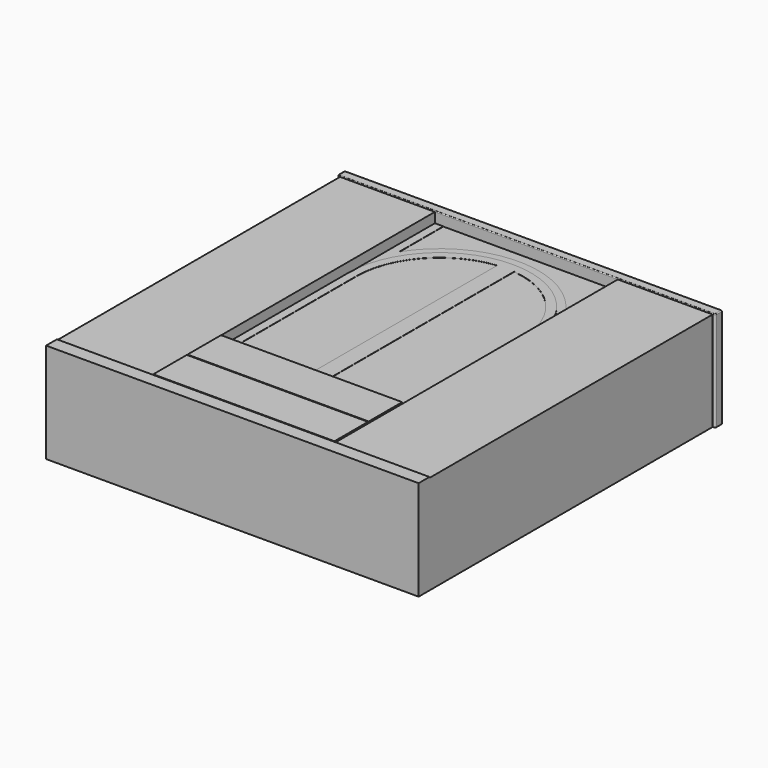
from build123d import *

# Parameters (mm, degrees)
F0_W     = 1070
F0_H     = 247.5
F0_W_2   = 440
F0_H_2   = 876.6265964508
F1_DEPTH = 590
F2_R     = 10
F3_DEPTH = 65
F4_DEPTH = 64
F5_DEPTH = 62
F6_DEPTH = 63
F7_DEPTH = 5
F8_R     = 4.99999
F9_DEPTH = 18


# Not quite as in the source:
# - a fillet or chamfer is up to 0.001 mm smaller than in the source, because OpenCascade refuses the exact size
# - a feature of the source that left no trace in its solid (it failed there, or was rolled back) is left out


with BuildPart() as f1:
    # F0 (on Top) → F1 (new body)
    with BuildSketch(Plane.XY):
        with BuildLine():
            Line((-1640, 1530), (-1640, 1135))
            Line((-1640, 1135), (-1640, 590))
            Line((-1640, 590), (-1100, 590))
            Line((-1100, 590), (-1100, 1511.6265964508))
            Line((-1100, 1511.6265964508), (-1100, 2020))
            Line((-1100, 2020), (-1100, 2070))
            ThreePointArc((-1100, 2070), (-1481.8376618407, 1911.8376618407), (-1640, 1530))
        make_face()
        with BuildLine():
            Line((-1150, 1530), (-1150, 1511.6265964508))
            Line((-1150, 1511.6265964508), (-1150, 635))
            Line((-1150, 635), (-1590, 635))
            Line((-1590, 635), (-1590, 1511.6265964508))
            Line((-1590, 1511.6265964508), (-1590, 1530))
            ThreePointArc((-1590, 1530), (-1463.7306695895, 1858.3291031876), (-1150, 2017.4423042782))
            Line((-1150, 2017.4423042782), (-1150, 1530))
        make_face(mode=Mode.SUBTRACT)
        with BuildLine():
            Line((-560, 590), (-560, 1135))
            Line((-560, 1135), (-560, 1530))
            ThreePointArc((-560, 1530), (-644.9475295345, 1820.7357032139), (-873.0638856418, 2020))
            Line((-873.0638856418, 2020), (-1100, 2020))
            Line((-1100, 2020), (-1100, 1511.6265964508))
            Line((-1100, 1511.6265964508), (-1100, 590))
            Line((-1100, 590), (-560, 590))
        make_face()
        with BuildLine():
            Line((-1050, 635), (-1050, 1511.6265964508))
            Line((-1050, 1511.6265964508), (-1050, 1530))
            Line((-1050, 1530), (-1050, 2017.4423042782))
            ThreePointArc((-1050, 2017.4423042782), (-736.2693304105, 1858.3291031876), (-610, 1530))
            Line((-610, 1530), (-610, 1511.6265964508))
            Line((-610, 1511.6265964508), (-610, 635))
            Line((-610, 635), (-1050, 635))
        make_face(mode=Mode.SUBTRACT)
        Polygon((-560, 80), (0, 80), (0, 1135), (-560, 1135), (-560, 590), align=None)
        Polygon((-2200, 1135), (-2200, 80), (-1640, 80), (-1640, 590), (-1640, 1135), align=None)
        Polygon((-2200, 2170), (-2200, 1135), (-1640, 1135), (-1640, 1530), (-1640, 2170), align=None)
        Polygon((-560, 1135), (0, 1135), (0, 2170), (-560, 2170), (-560, 1530), align=None)
        Polygon((-1100, 80), (-560, 80), (-560, 590), (-1100, 590), (-1640, 590), (-1640, 80), align=None)
        with Locations((-1100, 208.75)):
            Rectangle(F0_W, F0_H, mode=Mode.SUBTRACT)
        with Locations((-1100, 461.25)):
            Rectangle(F0_W, F0_H, mode=Mode.SUBTRACT)
        with Locations((-830, 1073.3132982254)):
            Rectangle(F0_W_2, F0_H_2)
        with Locations((-1370, 1073.3132982254)):
            Rectangle(F0_W_2, F0_H_2)
        with Locations((-1100, 461.25)):
            Rectangle(F0_W, F0_H)
        with Locations((-1100, 208.75)):
            Rectangle(F0_W, F0_H)
        Polygon((-2200, 0), (0, 0), (0, 80), (-560, 80), (-1100, 80), (-1640, 80), (-2200, 80), align=None)
        with BuildLine():
            Line((-1590, 1511.6265964508), (-1150, 1511.6265964508))
            Line((-1150, 1511.6265964508), (-1150, 1530))
            Line((-1150, 1530), (-1150, 2017.4423042782))
            ThreePointArc((-1150, 2017.4423042782), (-1463.7306695895, 1858.3291031876), (-1590, 1530))
            Line((-1590, 1530), (-1590, 1511.6265964508))
        make_face()
        with BuildLine():
            Line((-1050, 1530), (-1050, 1511.6265964508))
            Line((-1050, 1511.6265964508), (-610, 1511.6265964508))
            Line((-610, 1511.6265964508), (-610, 1530))
            ThreePointArc((-610, 1530), (-736.2693304105, 1858.3291031876), (-1050, 2017.4423042782))
            Line((-1050, 2017.4423042782), (-1050, 1530))
        make_face()
        Polygon((-560, 2170), (0, 2170), (15, 2170), (15, 2220), (0, 2220), (-2200, 2220), (-2215, 2220), (-2215, 2170), (-2200, 2170), (-1640, 2170), (-1590, 2170), (-1100, 2170), (-610, 2170), align=None)
        with BuildLine():
            Line((-1100, 2170), (-1590, 2170))
            Line((-1590, 2170), (-1590, 1846.2193073328))
            ThreePointArc((-1590, 1846.2193073328), (-1379.000923117, 2042.1065662827), (-1100, 2113.1763458252))
            Line((-1100, 2113.1763458252), (-1100, 2170))
        make_face()
        with BuildLine():
            Line((-610, 2020), (-610, 2170))
            Line((-610, 2170), (-1100, 2170))
            Line((-1100, 2170), (-1100, 2113.1763458252))
            ThreePointArc((-1100, 2113.1763458252), (-935.1694189847, 2089.397470402), (-783.7806926672, 2020))
            Line((-783.7806926672, 2020), (-610, 2020))
        make_face()
        with BuildLine():
            Line((-1590, 2170), (-1640, 2170))
            Line((-1640, 2170), (-1640, 1530))
            ThreePointArc((-1640, 1530), (-1481.8376618407, 1911.8376618407), (-1100, 2070))
            Line((-1100, 2070), (-1100, 2113.1763458252))
            ThreePointArc((-1100, 2113.1763458252), (-1379.000923117, 2042.1065662827), (-1590, 1846.2193073328))
            Line((-1590, 1846.2193073328), (-1590, 2170))
        make_face()
        with BuildLine():
            Line((-560, 1530), (-560, 2170))
            Line((-560, 2170), (-610, 2170))
            Line((-610, 2170), (-610, 2020))
            Line((-610, 2020), (-610, 1846.2193073328))
            ThreePointArc((-610, 1846.2193073328), (-687.6320512394, 1942.3679487606), (-783.7806926672, 2020))
            Line((-783.7806926672, 2020), (-873.0638856418, 2020))
            ThreePointArc((-873.0638856418, 2020), (-644.9475295345, 1820.7357032139), (-560, 1530))
        make_face()
        with BuildLine():
            Line((-610, 1846.2193073328), (-610, 2020))
            Line((-610, 2020), (-783.7806926672, 2020))
            ThreePointArc((-783.7806926672, 2020), (-687.6320512394, 1942.3679487606), (-610, 1846.2193073328))
        make_face()
        with BuildLine():
            ThreePointArc((-1100, 2070), (-983.8104996138, 2057.3518749374), (-873.0638856418, 2020))
            Line((-873.0638856418, 2020), (-783.7806926672, 2020))
            ThreePointArc((-783.7806926672, 2020), (-935.1694189847, 2089.397470402), (-1100, 2113.1763458252))
            Line((-1100, 2113.1763458252), (-1100, 2070))
        make_face()
        with BuildLine():
            Line((-1100, 2020), (-873.0638856418, 2020))
            ThreePointArc((-873.0638856418, 2020), (-983.8104996138, 2057.3518749374), (-1100, 2070))
            Line((-1100, 2070), (-1100, 2020))
        make_face()
    extrude(amount=-F1_DEPTH)

    # F2
    f2_edges = [f1.edges().sort_by_distance(p)[0] for p in [
        (15, 2170, -295),
        (-2215, 2170, -295),
    ]]
    fillet(f2_edges, radius=F2_R)

    # F0 (on Top) → F3 (cut)
    with BuildSketch(Plane.XY):
        with BuildLine():
            Line((-1100, 2170), (-1590, 2170))
            Line((-1590, 2170), (-1590, 1846.2193073328))
            ThreePointArc((-1590, 1846.2193073328), (-1379.000923117, 2042.1065662827), (-1100, 2113.1763458252))
            Line((-1100, 2113.1763458252), (-1100, 2170))
        make_face()
        with BuildLine():
            Line((-610, 2020), (-610, 2170))
            Line((-610, 2170), (-1100, 2170))
            Line((-1100, 2170), (-1100, 2113.1763458252))
            ThreePointArc((-1100, 2113.1763458252), (-935.1694189847, 2089.397470402), (-783.7806926672, 2020))
            Line((-783.7806926672, 2020), (-610, 2020))
        make_face()
        with BuildLine():
            Line((-610, 1846.2193073328), (-610, 2020))
            Line((-610, 2020), (-783.7806926672, 2020))
            ThreePointArc((-783.7806926672, 2020), (-687.6320512394, 1942.3679487606), (-610, 1846.2193073328))
        make_face()
    extrude(amount=-F3_DEPTH, mode=Mode.SUBTRACT)

    # F0 (on Top) → F4 (cut)
    with BuildSketch(Plane.XY):
        with BuildLine():
            Line((-1590, 2170), (-1640, 2170))
            Line((-1640, 2170), (-1640, 1530))
            ThreePointArc((-1640, 1530), (-1481.8376618407, 1911.8376618407), (-1100, 2070))
            Line((-1100, 2070), (-1100, 2113.1763458252))
            ThreePointArc((-1100, 2113.1763458252), (-1379.000923117, 2042.1065662827), (-1590, 1846.2193073328))
            Line((-1590, 1846.2193073328), (-1590, 2170))
        make_face()
        with BuildLine():
            ThreePointArc((-1100, 2070), (-983.8104996138, 2057.3518749374), (-873.0638856418, 2020))
            Line((-873.0638856418, 2020), (-783.7806926672, 2020))
            ThreePointArc((-783.7806926672, 2020), (-935.1694189847, 2089.397470402), (-1100, 2113.1763458252))
            Line((-1100, 2113.1763458252), (-1100, 2070))
        make_face()
        with BuildLine():
            Line((-560, 1530), (-560, 2170))
            Line((-560, 2170), (-610, 2170))
            Line((-610, 2170), (-610, 2020))
            Line((-610, 2020), (-610, 1846.2193073328))
            ThreePointArc((-610, 1846.2193073328), (-687.6320512394, 1942.3679487606), (-783.7806926672, 2020))
            Line((-783.7806926672, 2020), (-873.0638856418, 2020))
            ThreePointArc((-873.0638856418, 2020), (-644.9475295345, 1820.7357032139), (-560, 1530))
        make_face()
    extrude(amount=-F4_DEPTH, mode=Mode.SUBTRACT)

    # F0 (on Top) → F5 (cut)
    with BuildSketch(Plane.XY):
        with BuildLine():
            Line((-1640, 1530), (-1640, 1135))
            Line((-1640, 1135), (-1640, 590))
            Line((-1640, 590), (-1100, 590))
            Line((-1100, 590), (-1100, 1511.6265964508))
            Line((-1100, 1511.6265964508), (-1100, 2020))
            Line((-1100, 2020), (-1100, 2070))
            ThreePointArc((-1100, 2070), (-1481.8376618407, 1911.8376618407), (-1640, 1530))
        make_face()
        with BuildLine():
            Line((-1150, 1530), (-1150, 1511.6265964508))
            Line((-1150, 1511.6265964508), (-1150, 635))
            Line((-1150, 635), (-1590, 635))
            Line((-1590, 635), (-1590, 1511.6265964508))
            Line((-1590, 1511.6265964508), (-1590, 1530))
            ThreePointArc((-1590, 1530), (-1463.7306695895, 1858.3291031876), (-1150, 2017.4423042782))
            Line((-1150, 2017.4423042782), (-1150, 1530))
        make_face(mode=Mode.SUBTRACT)
        with BuildLine():
            Line((-1100, 2020), (-873.0638856418, 2020))
            ThreePointArc((-873.0638856418, 2020), (-983.8104996138, 2057.3518749374), (-1100, 2070))
            Line((-1100, 2070), (-1100, 2020))
        make_face()
        with BuildLine():
            Line((-560, 590), (-560, 1135))
            Line((-560, 1135), (-560, 1530))
            ThreePointArc((-560, 1530), (-644.9475295345, 1820.7357032139), (-873.0638856418, 2020))
            Line((-873.0638856418, 2020), (-1100, 2020))
            Line((-1100, 2020), (-1100, 1511.6265964508))
            Line((-1100, 1511.6265964508), (-1100, 590))
            Line((-1100, 590), (-560, 590))
        make_face()
        with BuildLine():
            Line((-1050, 635), (-1050, 1511.6265964508))
            Line((-1050, 1511.6265964508), (-1050, 1530))
            Line((-1050, 1530), (-1050, 2017.4423042782))
            ThreePointArc((-1050, 2017.4423042782), (-736.2693304105, 1858.3291031876), (-610, 1530))
            Line((-610, 1530), (-610, 1511.6265964508))
            Line((-610, 1511.6265964508), (-610, 635))
            Line((-610, 635), (-1050, 635))
        make_face(mode=Mode.SUBTRACT)
    extrude(amount=-F5_DEPTH, mode=Mode.SUBTRACT)

    # F0 (on Top) → F6 (cut)
    with BuildSketch(Plane.XY):
        with Locations((-1370, 1073.3132982254)):
            Rectangle(F0_W_2, F0_H_2)
        with Locations((-830, 1073.3132982254)):
            Rectangle(F0_W_2, F0_H_2)
        with BuildLine():
            Line((-1050, 1530), (-1050, 1511.6265964508))
            Line((-1050, 1511.6265964508), (-610, 1511.6265964508))
            Line((-610, 1511.6265964508), (-610, 1530))
            ThreePointArc((-610, 1530), (-736.2693304105, 1858.3291031876), (-1050, 2017.4423042782))
            Line((-1050, 2017.4423042782), (-1050, 1530))
        make_face()
        with BuildLine():
            Line((-1590, 1511.6265964508), (-1150, 1511.6265964508))
            Line((-1150, 1511.6265964508), (-1150, 1530))
            Line((-1150, 1530), (-1150, 2017.4423042782))
            ThreePointArc((-1150, 2017.4423042782), (-1463.7306695895, 1858.3291031876), (-1590, 1530))
            Line((-1590, 1530), (-1590, 1511.6265964508))
        make_face()
    extrude(amount=-F6_DEPTH, mode=Mode.SUBTRACT)

    # F0 (on Top) → F7 (cut)
    with BuildSketch(Plane.XY):
        Polygon((-2200, 2170), (-2200, 1135), (-1640, 1135), (-1640, 1530), (-1640, 2170), align=None)
        Polygon((-2200, 1135), (-2200, 80), (-1640, 80), (-1640, 590), (-1640, 1135), align=None)
        Polygon((-560, 1135), (0, 1135), (0, 2170), (-560, 2170), (-560, 1530), align=None)
        Polygon((-560, 80), (0, 80), (0, 1135), (-560, 1135), (-560, 590), align=None)
    extrude(amount=-F7_DEPTH, mode=Mode.SUBTRACT)

    # F8 (radius 5 in the source; OpenCascade refuses exactly that, so slightly less here)
    f8_edges = [f1.edges().sort_by_distance(p)[0] for p in [
        (-1100, 2170, 0),
    ]]
    fillet(f8_edges, radius=F8_R)

    # F0 (on Top) → F9 (cut)
    with BuildSketch(Plane.XY):
        Polygon((-1100, 80), (-560, 80), (-560, 590), (-1100, 590), (-1640, 590), (-1640, 80), align=None)
        with Locations((-1100, 208.75)):
            Rectangle(F0_W, F0_H, mode=Mode.SUBTRACT)
        with Locations((-1100, 461.25)):
            Rectangle(F0_W, F0_H, mode=Mode.SUBTRACT)
    extrude(amount=-F9_DEPTH, mode=Mode.SUBTRACT)


solid = f1.part
